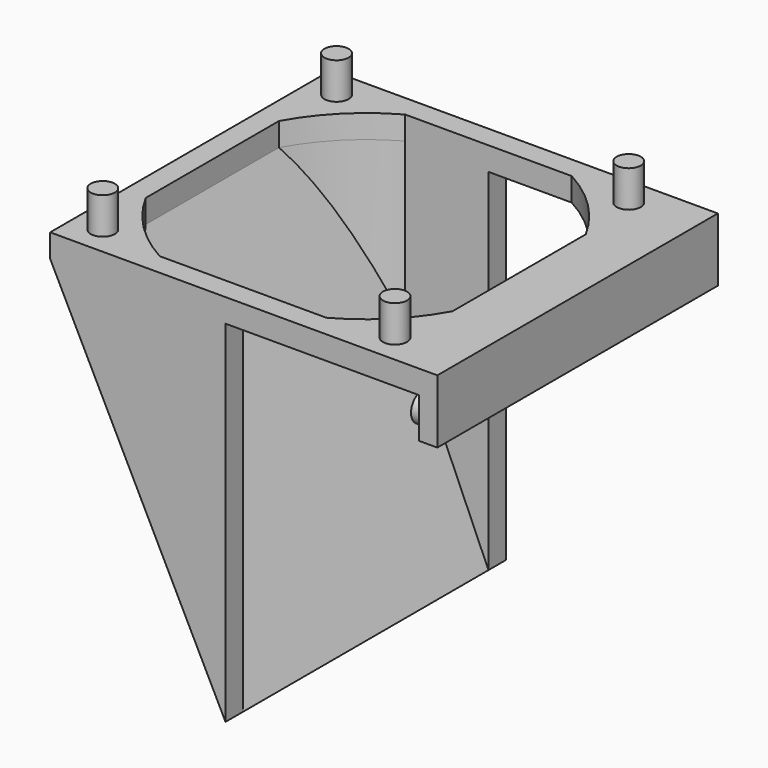
from build123d import *

# Parameters (mm, degrees)
F0_W        = 60.96
F0_H        = 4.064
F1_DEPTH    = 60.96
F3_DEPTH    = 25.4
F4_R        = 2.0955
F5_DEPTH    = 6.35
F7_DEPTH    = 60.96
F8_T4_DEPTH = 53.34
F8_S5_R     = 30.988
F8_T6_DEPTH = 44
F8_S7_R     = 30.48
F8_T8_DEPTH = 44
F9_W        = 60.96
F9_H        = 4.064
F10_DEPTH   = 6.35
F11_W       = 3.175
F11_H       = 60.96
F12_DEPTH   = 7
F13_R       = 2.5
F14_DEPTH   = 3
F15_R       = 2.5
F16_DEPTH   = 3


# Not quite as in the source:
# - a fillet or chamfer that OpenCascade refuses, or shapes differently, is made with other operations: its cross-section is extruded or revolved along the edge and cut away or added


with BuildPart() as f1:
    # F0 (on Right) → F1 (new body)
    with BuildSketch(Plane.YZ):
        with Locations((2.5902520865, 22.5415869818)):
            Rectangle(F0_W, F0_H)
    extrude(amount=F1_DEPTH)

    # F2 (on face) → F3 (cut)
    with BuildSketch(Plane.XY.offset(24.5735869818)):
        with BuildLine():
            Line((16.002, -24.0797479135), (44.958, -24.0797479135))
            ThreePointArc((44.958, -24.0797479135), (51.934072902, -18.8638208155), (57.15, -11.8877479135))
            Line((57.15, -11.8877479135), (57.15, 17.0682520865))
            ThreePointArc((57.15, 17.0682520865), (51.934072902, 24.0443249885), (44.958, 29.2602520865))
            Line((44.958, 29.2602520865), (16.002, 29.2602520865))
            ThreePointArc((16.002, 29.2602520865), (9.0409528702, 24.0292992163), (3.81, 17.0682520865))
            Line((3.81, 17.0682520865), (3.81, -11.8877479135))
            ThreePointArc((3.81, -11.8877479135), (9.025927098, -18.8638208155), (16.002, -24.0797479135))
        make_face()
    extrude(amount=-F3_DEPTH, mode=Mode.SUBTRACT)

    # F4 (on face) → F5 (join)
    with BuildSketch(Plane.XY.offset(24.5735869818)):
        with Locations((55.88, -22.8097479135)):
            Circle(F4_R)
        with Locations((55.88, 27.9902520865)):
            Circle(F4_R)
        with Locations((5.08, -22.8097479135)):
            Circle(F4_R)
        with Locations((5.08, 27.9902520865)):
            Circle(F4_R)
    extrude(amount=F5_DEPTH)

    # F6 (on face) → F7 (join)
    with BuildSketch(Plane.XZ.offset(27.8897479135)):
        Polygon((30.48, -40.4504130182), (30.48, 20.5095869818), (0, 20.5095869818), align=None)
    extrude(amount=-F7_DEPTH)

    # F8: chamfer of 60.96 x 26.67 on 1 edges, made by hand


with BuildPart() as f8_tool2:
    # F8_s3 → F8_t4 (new body)
    with BuildSketch(Plane.XZ.offset(24.0797479135)):
        Polygon((3.81, 20.5095869818), (30.48, -40.4504130182), (30.48, 20.5095869818), align=None)
    extrude(amount=-F8_T4_DEPTH)

    # F8_s5 → F8_t6 (intersect, symmetric)
    with BuildSketch(Plane.XY.offset(-10)):
        with Locations((30.9527778056, 2.1174742809)):
            Circle(F8_S5_R)
    extrude(amount=F8_T6_DEPTH, both=True, mode=Mode.INTERSECT)

    # F8_s7 → F8_t8 (intersect, symmetric)
    with BuildSketch(Plane.XY.offset(-10)):
        with Locations((30.5785417886, 2.6887938751)):
            Circle(F8_S7_R)
    extrude(amount=F8_T8_DEPTH, both=True, mode=Mode.INTERSECT)


with BuildPart() as f1_1:
    add(f1.part)

    # F8_t1: cut F8_tool2
    add(f8_tool2.part, mode=Mode.SUBTRACT)

    # F9 (on face) → F10 (join)
    with BuildSketch(Plane.YZ.offset(60.96)):
        with Locations((2.5902520865, 22.5415869818)):
            Rectangle(F9_W, F9_H)
    extrude(amount=F10_DEPTH)

    # F11 (on face) → F12 (join)
    with BuildSketch(Plane(origin=(0, 0, 20.5095869818), x_dir=(1, 0, 0), z_dir=(0, 0, -1))):
        with Locations((65.7225, -2.5902520865)):
            Rectangle(F11_W, F11_H)
    extrude(amount=F12_DEPTH)

    # F13 (on face) → F14 (join)
    with BuildSketch(Plane(origin=(64.135, 0, 0), x_dir=(0, -1, 0), z_dir=(-1, 0, 0))):
        with Locations((-28.5702520865, 16.0095869818)):
            Circle(F13_R)
    extrude(amount=F14_DEPTH)

    # F15 (on face) → F16 (join)
    with BuildSketch(Plane(origin=(64.135, 0, 0), x_dir=(0, -1, 0), z_dir=(-1, 0, 0))):
        with Locations((23.3897479135, 16.0095869818)):
            Circle(F15_R)
    extrude(amount=F16_DEPTH)


solid = f1_1.part
